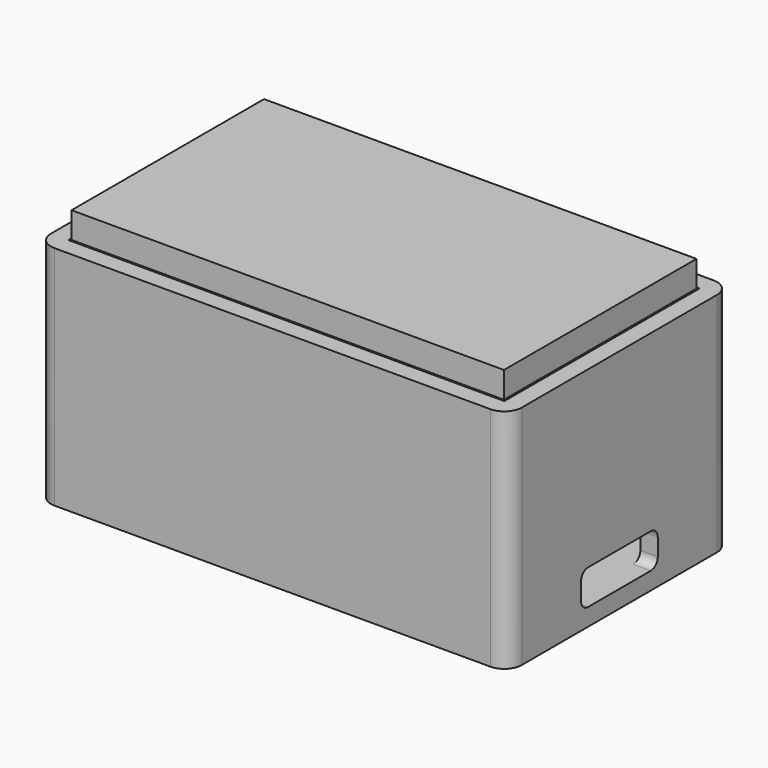
from build123d import *

# Parameters (mm, degrees)
F1_W      = 50
F1_H      = 28
F1_R      = 1.25
F2_DEPTH  = 24
F3_T      = 2
F4_DEPTH  = 15
F5_R      = 2
F6_W      = 11
F6_H      = 4
F7_DEPTH  = 2
F8_R      = 1
F9_W      = 49.6
F9_H      = 27.6
F9_R      = 1.45
F10_DEPTH = 3
F11_DEPTH = 1


with BuildPart() as f2:
    # F1 (on Top) → F2 (new body)
    with BuildSketch(Plane.XY):
        with Locations((1.0603448276, 0)):
            Rectangle(F1_W, F1_H)
        with Locations((-20.7396551724, -10.8)):
            Circle(F1_R, mode=Mode.SUBTRACT)
        with Locations((22.8603448276, -10.8)):
            Circle(F1_R, mode=Mode.SUBTRACT)
        with Locations((-20.7396551724, 10.8)):
            Circle(F1_R, mode=Mode.SUBTRACT)
        with Locations((22.8603448276, 10.8)):
            Circle(F1_R, mode=Mode.SUBTRACT)
        with Locations((22.8603448276, -10.8)):
            Circle(F1_R)
        with Locations((-20.7396551724, -10.8)):
            Circle(F1_R)
        with Locations((-20.7396551724, 10.8)):
            Circle(F1_R)
        with Locations((22.8603448276, 10.8)):
            Circle(F1_R)
    extrude(amount=F2_DEPTH)

    # F3
    f3_openings = [f2.faces().sort_by_distance(p)[0] for p in [
        (1.060345, 0, 24),
    ]]
    offset(amount=F3_T, openings=f3_openings, kind=Kind.INTERSECTION)

    # F1 (on Top) → F4 (join)
    with BuildSketch(Plane.XY):
        with Locations((-20.7396551724, -10.8)):
            Circle(F1_R)
        with Locations((-20.7396551724, 10.8)):
            Circle(F1_R)
        with Locations((22.8603448276, -10.8)):
            Circle(F1_R)
        with Locations((22.8603448276, 10.8)):
            Circle(F1_R)
    extrude(amount=F4_DEPTH)

    # F5
    f5_edges = [f2.edges().sort_by_distance(p)[0] for p in [
        (28.060345, -16, 11),
        (-25.939655, -16, 11),
        (28.060345, 16, 11),
        (-25.939655, 16, 11),
    ]]
    fillet(f5_edges, radius=F5_R)

    # F6 (on face) → F7 (cut)
    with BuildSketch(Plane.YZ.offset(28.0603448276)):
        with Locations((0, 2)):
            Rectangle(F6_W, F6_H)
    extrude(amount=-F7_DEPTH, mode=Mode.SUBTRACT)

    # F8
    f8_edges = [f2.edges().sort_by_distance(p)[0] for p in [
        (27.060345, 5.5, 4),
        (27.060345, -5.5, 4),
        (27.060345, 5.5, 0),
        (27.060345, -5.5, 0),
    ]]
    fillet(f8_edges, radius=F8_R)


with BuildPart() as f10:
    # F9 (on face) → F10 (new body)
    with BuildSketch(Plane.XY.offset(24)):
        with Locations((1.0603448276, 0)):
            Rectangle(F9_W, F9_H)
        with Locations((-20.7396551724, -10.8)):
            Circle(F9_R, mode=Mode.SUBTRACT)
        with Locations((22.8603448276, -10.8)):
            Circle(F9_R, mode=Mode.SUBTRACT)
        with Locations((-20.7396551724, 10.8)):
            Circle(F9_R, mode=Mode.SUBTRACT)
        with Locations((22.8603448276, 10.8)):
            Circle(F9_R, mode=Mode.SUBTRACT)
        with Locations((-20.7396551724, -10.8)):
            Circle(F9_R)
        with Locations((22.8603448276, -10.8)):
            Circle(F9_R)
        with Locations((22.8603448276, 10.8)):
            Circle(F9_R)
        with Locations((-20.7396551724, 10.8)):
            Circle(F9_R)
    extrude(amount=F10_DEPTH)

    # F9 (on face) → F11 (cut)
    with BuildSketch(Plane.XY.offset(24)):
        with Locations((-20.7396551724, -10.8)):
            Circle(F9_R)
        with Locations((-20.7396551724, 10.8)):
            Circle(F9_R)
        with Locations((22.8603448276, 10.8)):
            Circle(F9_R)
        with Locations((22.8603448276, -10.8)):
            Circle(F9_R)
    extrude(amount=F11_DEPTH, mode=Mode.SUBTRACT)


solid = Compound([f2.part, f10.part])
